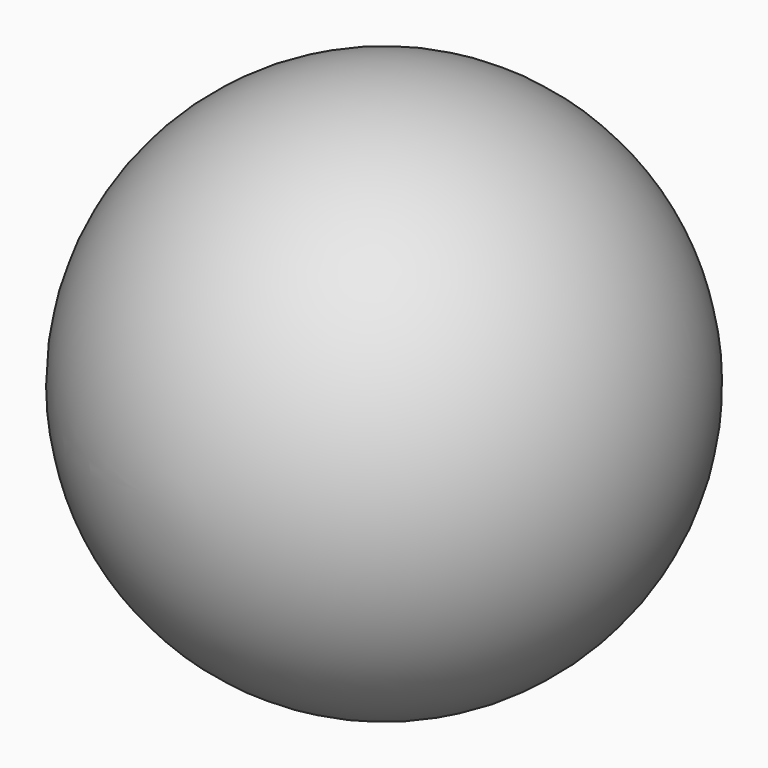
from build123d import *


# Not quite as in the source:
# - the program builds the solid bodies; features that only make, move or delete a surface that nothing else refers to are left out


with BuildPart() as f1:
    # F0 (on Top) → F1 (revolve)
    with BuildSketch(Plane.XY):
        with BuildLine():
            Line((0, -15.875), (0, 15.875))
            ThreePointArc((0, 15.875), (-15.875, 0), (0, -15.875))
        make_face()
    revolve(axis=Axis((0, 0, 0), (0, 1, 0)))


solid = f1.part
